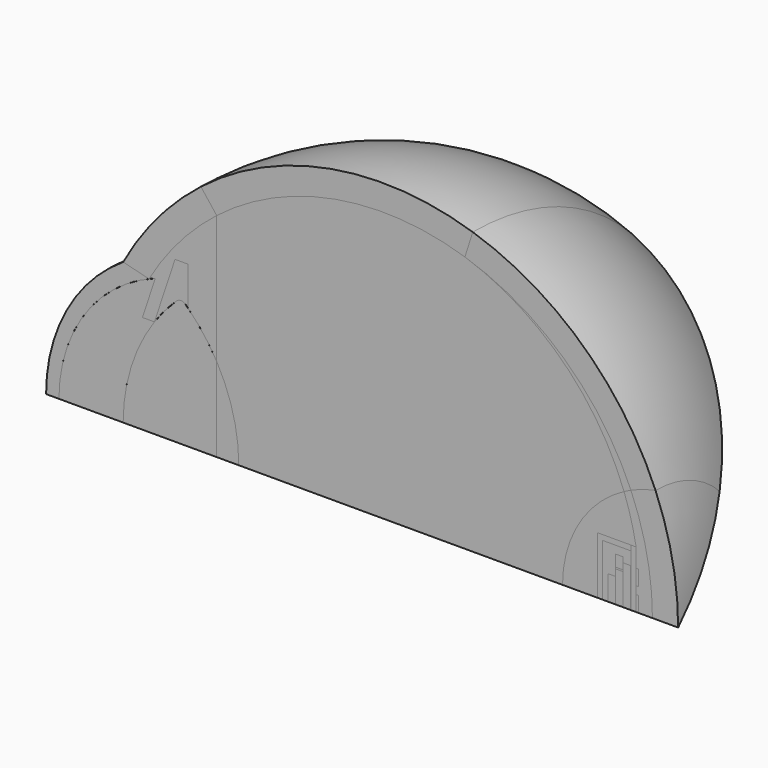
from build123d import *

# Parameters (mm, degrees)
F1_ANGLE  = 45
F3_ANGLE  = 45
F4_ANGLE  = 45
F6_ANGLE  = 45
F7_ANGLE  = 45
F9_ANGLE  = 45
F10_ANGLE = 45
F11_W     = 1.51221
F11_H     = 2.23
F12_ANGLE = 45
F13_ANGLE = 45
F15_ANGLE = 45
F16_ANGLE = 45
F19_ANGLE = 45
F22_ANGLE = 45
F25_ANGLE = 45
F28_ANGLE = 45
F31_ANGLE = 45
F34_ANGLE = 45
F35_W     = 0.19
F35_H     = 2.23
F36_ANGLE = 45
F37_W     = 0.19
F37_H     = 2.23
F38_ANGLE = 45
F40_ANGLE = 45
F41_ANGLE = 45
F42_W     = 0.3
F42_H     = 1.5222
F44_ANGLE = 45
F45_W     = 0.28
F45_H     = 1.2205
F47_ANGLE = 45
F48_W     = 0.301
F48_H     = 0.95912
F50_ANGLE = 45
F51_W     = 0.28
F51_H     = 0.447172
F53_ANGLE = 45
F54_W     = 0.025
F54_H     = 0.25075
F56_ANGLE = 45
F57_W     = 0.1
F57_H     = 0.6
F59_ANGLE = 45
F62_ANGLE = 45
F65_ANGLE = 45
F68_ANGLE = 45
F69_W     = 0.28
F69_H     = 0.06
F71_ANGLE = 45


with BuildPart() as f1:
    # F0 (on Front) → F1 (revolve)
    with BuildSketch(Plane.XZ):
        with BuildLine():
            Line((-11.5, 0), (11.5, 0))
            ThreePointArc((11.5, 0), (2.8377537956, 11.1443776585), (-10.0995049384, 5.5))
            ThreePointArc((-10.0995049384, 5.5), (-12.3007384778, 3.1324910215), (-13.0995049384, 0))
            Line((-13.0995049384, 0), (-11.5, 0))
        make_face()
    revolve(axis=Axis((0, 0, 0), (-1, 0, 0)), revolution_arc=F1_ANGLE)

    # F2 (on Front) → F3 (revolve, cut)
    with BuildSketch(Plane.XZ):
        with BuildLine():
            ThreePointArc((11.5, 0), (2.8377537956, 11.1443776585), (-10.0995049384, 5.5))
            Line((-10.0995049384, 5.5), (-9.0932667397, 5.25))
            ThreePointArc((-9.0932667397, 5.25), (2.7175999736, 10.142221176), (10.5, 0))
            Line((10.5, 0), (11.5, 0))
        make_face()
    revolve(axis=Axis((0, 0, 0), (-1, 0, 0)), revolution_arc=F3_ANGLE, mode=Mode.SUBTRACT)

    # F5 (on face) → F6 (revolve, cut)
    with BuildSketch(Plane.XZ):
        with BuildLine():
            ThreePointArc((-12.5995049384, 0), (-11.6423500551, 3.1565885979), (-9.0932667397, 5.25))
            Line((-9.0932667397, 5.25), (-10.0995049384, 5.5))
            ThreePointArc((-10.0995049384, 5.5), (-12.3007384778, 3.1324910215), (-13.0995049384, 0))
            Line((-13.0995049384, 0), (-12.5995049384, 0))
        make_face()
    revolve(axis=Axis((-12.2997524692, 0, 0), (-1, 0, 0)), revolution_arc=F6_ANGLE, mode=Mode.SUBTRACT)

    # F8 (on Front) → F9 (revolve, cut)
    with BuildSketch(Plane.XZ):
        with BuildLine():
            ThreePointArc((3.2015621187, 10), (8.2807192075, 6.1420955145), (10, 0))
            Line((10, 0), (10.5, 0))
            ThreePointArc((10.5, 0), (8.4813442993, 6.1900564518), (3.2015621187, 10))
        make_face()
    revolve(axis=Axis((0, 0, 0), (-1, 0, 0)), revolution_arc=F9_ANGLE, mode=Mode.SUBTRACT)

    # F11 (on face) → F12 (revolve, cut)
    with BuildSketch(Plane.XZ):
        with Locations((9.1086225685, 1.115)):
            Rectangle(F11_W, F11_H)
    revolve(axis=Axis((9.1086225685, 0, 0), (-1, 0, 0)), revolution_arc=F12_ANGLE, mode=Mode.SUBTRACT)

    # F14 (on Front) → F15 (revolve, cut)
    with BuildSketch(Plane.XZ):
        with BuildLine():
            ThreePointArc((10, 0), (9.9947523902, 1.1187845105), (9.8647275685, 2.23))
            Line((9.8647275685, 2.23), (9.8647275685, 0))
            Line((9.8647275685, 0), (10, 0))
        make_face()
    revolve(axis=Axis((9.9323637842, 0, 0), (-1, 0, 0)), revolution_arc=F15_ANGLE, mode=Mode.SUBTRACT)

    # F20 (on Front) → F21 (revolve, cut)
    with BuildSketch(Plane.XZ):
        with BuildLine():
            Line((-9.3495049384, 3.8445862413), (-8.8495049384, 5.3445862413))
            ThreePointArc((-8.8495049384, 5.3445862413), (-11.5684914777, 3.2644717065), (-12.5995049384, 0))
            Line((-12.5995049384, 0), (-8.8495049384, 0))
            Line((-8.8495049384, 0), (-8.8495049384, 3.8445862413))
            Line((-8.8495049384, 3.8445862413), (-9.3495049384, 3.8445862413))
        make_face()
    revolve(axis=Axis((-10.7245049384, 0, 0), (1, 0, 0)), mode=Mode.SUBTRACT)


with BuildPart() as f4:
    # F2 (on Front) → F4 (revolve)
    with BuildSketch(Plane.XZ):
        with BuildLine():
            ThreePointArc((11.5, 0), (2.8377537956, 11.1443776585), (-10.0995049384, 5.5))
            Line((-10.0995049384, 5.5), (-9.0932667397, 5.25))
            ThreePointArc((-9.0932667397, 5.25), (2.7175999736, 10.142221176), (10.5, 0))
            Line((10.5, 0), (11.5, 0))
        make_face()
    revolve(axis=Axis((0, 0, 0), (-1, 0, 0)), revolution_arc=F4_ANGLE)

    # F17 (on Front) → F18 (revolve, cut)
    with BuildSketch(Plane.XZ):
        with BuildLine():
            ThreePointArc((11.5, 0), (9.2890913754, 6.7795856377), (3.5064727967, 10.9523809524))
            Line((3.5064727967, 10.9523809524), (3.2015621187, 10))
            ThreePointArc((3.2015621187, 10), (8.4813442993, 6.1900564518), (10.5, 0))
            Line((10.5, 0), (11.5, 0))
        make_face()
    revolve(axis=Axis((11, 0, 0), (1, 0, 0)), mode=Mode.SUBTRACT)

    # F29 (on Front) → F30 (revolve, cut)
    with BuildSketch(Plane.XZ):
        with BuildLine():
            ThreePointArc((-9.0932667397, 5.25), (-7.9222484154, 6.8911523017), (-6.4591549508, 8.2782436134))
            Line((-6.4591549508, 8.2782436134), (-7.0743125651, 9.066647767))
            ThreePointArc((-7.0743125651, 9.066647767), (-8.7701337495, 7.438733361), (-10.0995049384, 5.5))
            Line((-10.0995049384, 5.5), (-9.0932667397, 5.25))
        make_face()
    revolve(axis=Axis((-7.8495049384, 0, 0), (-1, 0, 0)), mode=Mode.SUBTRACT)


with BuildPart() as f7:
    # F5 (on face) → F7 (revolve)
    with BuildSketch(Plane.XZ):
        with BuildLine():
            ThreePointArc((-12.5995049384, 0), (-11.6423500551, 3.1565885979), (-9.0932667397, 5.25))
            Line((-9.0932667397, 5.25), (-10.0995049384, 5.5))
            ThreePointArc((-10.0995049384, 5.5), (-12.3007384778, 3.1324910215), (-13.0995049384, 0))
            Line((-13.0995049384, 0), (-12.5995049384, 0))
        make_face()
    revolve(axis=Axis((0, 0, 0), (-1, 0, 0)), revolution_arc=F7_ANGLE)


with BuildPart() as f10:
    # F8 (on Front) → F10 (revolve)
    with BuildSketch(Plane.XZ):
        with BuildLine():
            ThreePointArc((3.2015621187, 10), (8.2807192075, 6.1420955145), (10, 0))
            Line((10, 0), (10.5, 0))
            ThreePointArc((10.5, 0), (8.4813442993, 6.1900564518), (3.2015621187, 10))
        make_face()
    revolve(axis=Axis((10.25, 0, 0), (-1, 0, 0)), revolution_arc=F10_ANGLE)


with BuildPart() as f13:
    # F11 (on face) → F13 (revolve)
    with BuildSketch(Plane.XZ):
        with Locations((9.1086225685, 1.115)):
            Rectangle(F11_W, F11_H)
    revolve(axis=Axis((0, 0, 0), (-1, 0, 0)), revolution_arc=F13_ANGLE)

    # F35 (on face) → F36 (revolve, cut)
    with BuildSketch(Plane.XZ):
        with Locations((9.7697275685, 1.115)):
            Rectangle(F35_W, F35_H)
    revolve(axis=Axis((0, 0, 0), (-1, 0, 0)), revolution_arc=F36_ANGLE, mode=Mode.SUBTRACT)

    # F39 (on face) → F40 (revolve, cut)
    with BuildSketch(Plane.XZ):
        Polygon((8.3525175685, 0), (8.5525175685, 0), (8.5525175685, 2.03), (9.6747275685, 2.03), (9.6747275685, 2.23), (8.3525175685, 2.23), align=None)
    revolve(axis=Axis((0, 0, 0), (-1, 0, 0)), revolution_arc=F40_ANGLE, mode=Mode.SUBTRACT)

    # F42 (on face) → F43 (revolve, cut)
    with BuildSketch(Plane.XZ):
        with Locations((9.4997275685, 0.7611)):
            Rectangle(F42_W, F42_H)
    revolve(axis=Axis((9.4997275685, 0, 0), (-1, 0, 0)), mode=Mode.SUBTRACT)

    # F45 (on face) → F46 (revolve, cut)
    with BuildSketch(Plane.XZ):
        with Locations((9.2097275685, 0.61025)):
            Rectangle(F45_W, F45_H)
    revolve(axis=Axis((9.2097275685, 0, 0), (-1, 0, 0)), mode=Mode.SUBTRACT)

    # F48 (on face) → F49 (revolve, cut)
    with BuildSketch(Plane.XZ):
        with Locations((8.9192275685, 0.47956)):
            Rectangle(F48_W, F48_H)
    revolve(axis=Axis((8.9192275685, 0, 0), (-1, 0, 0)), mode=Mode.SUBTRACT)

    # F51 (on face) → F52 (revolve, cut)
    with BuildSketch(Plane.XZ):
        with Locations((9.2097275685, 1.504086)):
            Rectangle(F51_W, F51_H)
    revolve(axis=Axis((0, 0, 0), (-1, 0, 0)), mode=Mode.SUBTRACT)

    # F54 (on face) → F55 (revolve, cut)
    with BuildSketch(Plane.XZ):
        with Locations((9.6622275685, 0.125375)):
            Rectangle(F54_W, F54_H)
        with Locations((9.6622275685, 1.125375)):
            Rectangle(F54_W, F54_H)
    revolve(axis=Axis((9.6622275685, 0, 0), (-1, 0, 0)), mode=Mode.SUBTRACT)

    # F69 (on face) → F70 (revolve, cut)
    with BuildSketch(Plane.XZ):
        with Locations((9.2097275685, 1.2505)):
            Rectangle(F69_W, F69_H)
    revolve(axis=Axis((0, 0, 0), (-1, 0, 0)), mode=Mode.SUBTRACT)


with BuildPart() as f16:
    # F14 (on Front) → F16 (revolve)
    with BuildSketch(Plane.XZ):
        with BuildLine():
            ThreePointArc((10, 0), (9.9947523902, 1.1187845105), (9.8647275685, 2.23))
            Line((9.8647275685, 2.23), (9.8647275685, 0))
            Line((9.8647275685, 0), (10, 0))
        make_face()
    revolve(axis=Axis((0, 0, 0), (-1, 0, 0)), revolution_arc=F16_ANGLE)


with BuildPart() as f19:
    # F17 (on Front) → F19 (revolve)
    with BuildSketch(Plane.XZ):
        with BuildLine():
            ThreePointArc((11.5, 0), (9.2890913754, 6.7795856377), (3.5064727967, 10.9523809524))
            Line((3.5064727967, 10.9523809524), (3.2015621187, 10))
            ThreePointArc((3.2015621187, 10), (8.4813442993, 6.1900564518), (10.5, 0))
            Line((10.5, 0), (11.5, 0))
        make_face()
    revolve(axis=Axis((0, 0, 0), (-1, 0, 0)), revolution_arc=F19_ANGLE)

    # F63 (on face) → F64 (revolve, cut)
    with BuildSketch(Plane.XZ):
        with BuildLine():
            ThreePointArc((11.5, 0), (11.2777435686, 2.25), (10.6195652174, 4.4130300921))
            ThreePointArc((10.6195652174, 4.4130300921), (10.1327706577, 4.2872699851), (9.6630434783, 4.1079910829))
            ThreePointArc((9.6630434783, 4.1079910829), (10.2886334496, 2.0961921999), (10.5, 0))
            Line((10.5, 0), (11.5, 0))
        make_face()
    revolve(axis=Axis((11, 0, 0), (-1, 0, 0)), mode=Mode.SUBTRACT)


with BuildPart() as f22:
    # F20 (on Front) → F22 (revolve)
    with BuildSketch(Plane.XZ):
        with BuildLine():
            Line((-9.3495049384, 3.8445862413), (-8.8495049384, 5.3445862413))
            ThreePointArc((-8.8495049384, 5.3445862413), (-11.5684914777, 3.2644717065), (-12.5995049384, 0))
            Line((-12.5995049384, 0), (-8.8495049384, 0))
            Line((-8.8495049384, 0), (-8.8495049384, 3.8445862413))
            Line((-8.8495049384, 3.8445862413), (-9.3495049384, 3.8445862413))
        make_face()
    revolve(axis=Axis((0, 0, 0), (-1, 0, 0)), revolution_arc=F22_ANGLE)


with BuildPart() as f24_tool:
    # F23 (on Front) → F24 (revolve)
    with BuildSketch(Plane.XZ):
        with BuildLine():
            Line((-10.0995049384, 0), (-5.5995049384, 0))
            ThreePointArc((-5.5995049384, 0), (-6.1408791354, 2.6344401261), (-7.6772587181, 4.8419044128))
            ThreePointArc((-7.6772587181, 4.8419044128), (-7.8495049384, 4.9107104847), (-8.0217511587, 4.8419044128))
            ThreePointArc((-8.0217511587, 4.8419044128), (-9.5581307413, 2.6344401261), (-10.0995049384, 0))
        make_face()
    revolve(axis=Axis((0, 0, 0), (-1, 0, 0)))


with BuildPart() as f1_1:
    add(f1.part)

    # F24: cut by f24_tool
    add(f24_tool.part, mode=Mode.SUBTRACT)

    # F26 (on Front) → F27 (revolve, cut)
    with BuildSketch(Plane.XZ):
        with BuildLine():
            Line((-8.8495049384, 5.3445862413), (-9.3495049384, 3.8445862413))
            Line((-9.3495049384, 3.8445862413), (-8.8823713109, 3.8445862413))
            Line((-8.8823713109, 3.8445862413), (-8.0810395972, 6.2485813822))
            Line((-8.0810395972, 6.2485813822), (-7.5810395972, 6.2485813822))
            Line((-7.5810395972, 6.2485813822), (-7.5810395972, 4.7485813822))
            ThreePointArc((-7.5810395972, 4.7485813822), (-6.9689696113, 4.0524234931), (-6.4591549508, 3.2782436134))
            Line((-6.4591549508, 3.2782436134), (-6.4591549508, 8.2782436134))
            ThreePointArc((-6.4591549508, 8.2782436134), (-7.9222484154, 6.8911523017), (-9.0932667397, 5.25))
            ThreePointArc((-9.0932667397, 5.25), (-8.9719298306, 5.298695062), (-8.8495049384, 5.3445862413))
        make_face()
    revolve(axis=Axis((-7.8495049384, 0, 0), (-1, 0, 0)), mode=Mode.SUBTRACT)

    # F60 (on face) → F61 (revolve, cut)
    with BuildSketch(Plane.XZ):
        with BuildLine():
            ThreePointArc((9.8647275685, 2.23), (9.6692210389, 3.1141957451), (9.3946322021, 3.9771128266))
            ThreePointArc((9.3946322021, 3.9771128266), (7.6448634855, 2.3211898791), (7, 0))
            Line((7, 0), (8.3525175685, 0))
            Line((8.3525175685, 0), (8.3525175685, 2.23))
            Line((8.3525175685, 2.23), (9.8647275685, 2.23))
        make_face()
    revolve(axis=Axis((7.6762587842, 0, 0), (1, 0, 0)), mode=Mode.SUBTRACT)


with BuildPart() as f22_1:
    add(f22.part)

    # F24: cut by f24_tool
    add(f24_tool.part, mode=Mode.SUBTRACT)


with BuildPart() as f25:
    # F23 (on Front) → F25 (revolve)
    with BuildSketch(Plane.XZ):
        with BuildLine():
            Line((-10.0995049384, 0), (-5.5995049384, 0))
            ThreePointArc((-5.5995049384, 0), (-6.1408791354, 2.6344401261), (-7.6772587181, 4.8419044128))
            ThreePointArc((-7.6772587181, 4.8419044128), (-7.8495049384, 4.9107104847), (-8.0217511587, 4.8419044128))
            ThreePointArc((-8.0217511587, 4.8419044128), (-9.5581307413, 2.6344401261), (-10.0995049384, 0))
        make_face()
    revolve(axis=Axis((0, 0, 0), (-1, 0, 0)), revolution_arc=F25_ANGLE)

    # F32 (on Front) → F33 (revolve, cut)
    with BuildSketch(Plane.XZ):
        with BuildLine():
            Line((-6.4591549508, 3.2782436134), (-6.4591549508, 0))
            Line((-6.4591549508, 0), (-5.5995049384, 0))
            ThreePointArc((-5.5995049384, 0), (-5.8179901834, 1.6945411866), (-6.4591549508, 3.2782436134))
        make_face()
    revolve(axis=Axis((-6.0293299446, 0, 0), (1, 0, 0)), mode=Mode.SUBTRACT)


with BuildPart() as f28:
    # F26 (on Front) → F28 (revolve)
    with BuildSketch(Plane.XZ):
        with BuildLine():
            Line((-8.8495049384, 5.3445862413), (-9.3495049384, 3.8445862413))
            Line((-9.3495049384, 3.8445862413), (-8.8823713109, 3.8445862413))
            Line((-8.8823713109, 3.8445862413), (-8.0810395972, 6.2485813822))
            Line((-8.0810395972, 6.2485813822), (-7.5810395972, 6.2485813822))
            Line((-7.5810395972, 6.2485813822), (-7.5810395972, 4.7485813822))
            ThreePointArc((-7.5810395972, 4.7485813822), (-6.9689696113, 4.0524234931), (-6.4591549508, 3.2782436134))
            Line((-6.4591549508, 3.2782436134), (-6.4591549508, 8.2782436134))
            ThreePointArc((-6.4591549508, 8.2782436134), (-7.9222484154, 6.8911523017), (-9.0932667397, 5.25))
            ThreePointArc((-9.0932667397, 5.25), (-8.9719298306, 5.298695062), (-8.8495049384, 5.3445862413))
        make_face()
    revolve(axis=Axis((-7.8495049384, 0, 0), (-1, 0, 0)), revolution_arc=F28_ANGLE)


with BuildPart() as f31:
    # F29 (on Front) → F31 (revolve)
    with BuildSketch(Plane.XZ):
        with BuildLine():
            ThreePointArc((-9.0932667397, 5.25), (-7.9222484154, 6.8911523017), (-6.4591549508, 8.2782436134))
            Line((-6.4591549508, 8.2782436134), (-7.0743125651, 9.066647767))
            ThreePointArc((-7.0743125651, 9.066647767), (-8.7701337495, 7.438733361), (-10.0995049384, 5.5))
            Line((-10.0995049384, 5.5), (-9.0932667397, 5.25))
        make_face()
    revolve(axis=Axis((-7.8495049384, 0, 0), (-1, 0, 0)), revolution_arc=F31_ANGLE)


with BuildPart() as f34:
    # F32 (on Front) → F34 (revolve)
    with BuildSketch(Plane.XZ):
        with BuildLine():
            Line((-6.4591549508, 3.2782436134), (-6.4591549508, 0))
            Line((-6.4591549508, 0), (-5.5995049384, 0))
            ThreePointArc((-5.5995049384, 0), (-5.8179901834, 1.6945411866), (-6.4591549508, 3.2782436134))
        make_face()
    revolve(axis=Axis((-7.8495049384, 0, 0), (-1, 0, 0)), revolution_arc=F34_ANGLE)


with BuildPart() as f38:
    # F37 (on face) → F38 (revolve)
    with BuildSketch(Plane.XZ):
        with Locations((9.7697275685, 1.115)):
            Rectangle(F37_W, F37_H)
    revolve(axis=Axis((0, 0, 0), (-1, 0, 0)), revolution_arc=F38_ANGLE)


with BuildPart() as f41:
    # F39 (on face) → F41 (revolve)
    with BuildSketch(Plane.XZ):
        Polygon((8.3525175685, 0), (8.5525175685, 0), (8.5525175685, 2.03), (9.6747275685, 2.03), (9.6747275685, 2.23), (8.3525175685, 2.23), align=None)
    revolve(axis=Axis((0, 0, 0), (-1, 0, 0)), revolution_arc=F41_ANGLE)


with BuildPart() as f44:
    # F42 (on face) → F44 (revolve)
    with BuildSketch(Plane.XZ):
        with Locations((9.4997275685, 0.7611)):
            Rectangle(F42_W, F42_H)
    revolve(axis=Axis((0, 0, 0), (-1, 0, 0)), revolution_arc=F44_ANGLE)


with BuildPart() as f47:
    # F45 (on face) → F47 (revolve)
    with BuildSketch(Plane.XZ):
        with Locations((9.2097275685, 0.61025)):
            Rectangle(F45_W, F45_H)
    revolve(axis=Axis((0, 0, 0), (-1, 0, 0)), revolution_arc=F47_ANGLE)


with BuildPart() as f50:
    # F48 (on face) → F50 (revolve)
    with BuildSketch(Plane.XZ):
        with Locations((8.9192275685, 0.47956)):
            Rectangle(F48_W, F48_H)
    revolve(axis=Axis((0, 0, 0), (-1, 0, 0)), revolution_arc=F50_ANGLE)


with BuildPart() as f53:
    # F51 (on face) → F53 (revolve)
    with BuildSketch(Plane.XZ):
        with Locations((9.2097275685, 1.504086)):
            Rectangle(F51_W, F51_H)
    revolve(axis=Axis((0, 0, 0), (-1, 0, 0)), revolution_arc=F53_ANGLE)


with BuildPart() as f56:
    # F54 (on face) → F56 (revolve)
    with BuildSketch(Plane.XZ):
        with Locations((9.6622275685, 0.125375)):
            Rectangle(F54_W, F54_H)
    revolve(axis=Axis((0, 0, 0), (-1, 0, 0)), revolution_arc=F56_ANGLE)


with BuildPart() as f56b:
    # F54 (on face) → F56, piece 2 (revolve)
    with BuildSketch(Plane.XZ):
        with Locations((9.6622275685, 1.125375)):
            Rectangle(F54_W, F54_H)
    revolve(axis=Axis((0, 0, 0), (-1, 0, 0)), revolution_arc=F56_ANGLE)


with BuildPart() as f58_tool:
    # F57 (on face) → F58 (revolve)
    with BuildSketch(Plane.XZ):
        with Locations((9.9147275685, 0.3)):
            Rectangle(F57_W, F57_H)
        with Locations((9.9147275685, 1.2)):
            Rectangle(F57_W, F57_H)
    revolve(axis=Axis((9.9147275685, 0, 0), (1, 0, 0)))


with BuildPart() as f10_1:
    add(f10.part)

    # F58: cut by f58_tool
    add(f58_tool.part, mode=Mode.SUBTRACT)


with BuildPart() as f16_1:
    add(f16.part)

    # F58: cut by f58_tool
    add(f58_tool.part, mode=Mode.SUBTRACT)


with BuildPart() as f59:
    # F57 (on face) → F59 (revolve)
    with BuildSketch(Plane.XZ):
        with Locations((9.9147275685, 0.3)):
            Rectangle(F57_W, F57_H)
    revolve(axis=Axis((0, 0, 0), (-1, 0, 0)), revolution_arc=F59_ANGLE)


with BuildPart() as f59b:
    # F57 (on face) → F59, piece 2 (revolve)
    with BuildSketch(Plane.XZ):
        with Locations((9.9147275685, 1.2)):
            Rectangle(F57_W, F57_H)
    revolve(axis=Axis((0, 0, 0), (-1, 0, 0)), revolution_arc=F59_ANGLE)


with BuildPart() as f62:
    # F60 (on face) → F62 (revolve)
    with BuildSketch(Plane.XZ):
        with BuildLine():
            ThreePointArc((9.8647275685, 2.23), (9.6692210389, 3.1141957451), (9.3946322021, 3.9771128266))
            ThreePointArc((9.3946322021, 3.9771128266), (7.6448634855, 2.3211898791), (7, 0))
            Line((7, 0), (8.3525175685, 0))
            Line((8.3525175685, 0), (8.3525175685, 2.23))
            Line((8.3525175685, 2.23), (9.8647275685, 2.23))
        make_face()
    revolve(axis=Axis((0, 0, 0), (-1, 0, 0)), revolution_arc=F62_ANGLE)


with BuildPart() as f65:
    # F63 (on face) → F65 (revolve)
    with BuildSketch(Plane.XZ):
        with BuildLine():
            ThreePointArc((11.5, 0), (11.2777435686, 2.25), (10.6195652174, 4.4130300921))
            ThreePointArc((10.6195652174, 4.4130300921), (10.1327706577, 4.2872699851), (9.6630434783, 4.1079910829))
            ThreePointArc((9.6630434783, 4.1079910829), (10.2886334496, 2.0961921999), (10.5, 0))
            Line((10.5, 0), (11.5, 0))
        make_face()
    revolve(axis=Axis((0, 0, 0), (-1, 0, 0)), revolution_arc=F65_ANGLE)


with BuildPart() as f67_tool:
    # F66 (on face) → F67 (revolve)
    with BuildSketch(Plane.XZ):
        with BuildLine():
            ThreePointArc((10.5, 0), (10.2886334496, 2.0961921999), (9.6630434783, 4.1079910829))
            ThreePointArc((9.6630434783, 4.1079910829), (9.5277519071, 4.0447790372), (9.3946322021, 3.9771128266))
            ThreePointArc((9.3946322021, 3.9771128266), (9.6692210389, 3.1141957451), (9.8647275685, 2.23))
            Line((9.8647275685, 2.23), (9.8647275685, 1.5))
            Line((9.8647275685, 1.5), (9.9647275685, 1.5))
            Line((9.9647275685, 1.5), (9.9647275685, 0.9))
            Line((9.9647275685, 0.9), (9.8647275685, 0.9))
            Line((9.8647275685, 0.9), (9.8647275685, 0.6))
            Line((9.8647275685, 0.6), (9.9647275685, 0.6))
            Line((9.9647275685, 0.6), (9.9647275685, 0))
            Line((9.9647275685, 0), (10.5, 0))
        make_face()
    revolve(axis=Axis((10.2323637842, 0, 0), (-1, 0, 0)))


with BuildPart() as f10_2:
    add(f10_1.part)

    # F67: cut by f67_tool
    add(f67_tool.part, mode=Mode.SUBTRACT)


with BuildPart() as f16_2:
    add(f16_1.part)

    # F67: cut by f67_tool
    add(f67_tool.part, mode=Mode.SUBTRACT)


with BuildPart() as f68:
    # F66 (on face) → F68 (revolve)
    with BuildSketch(Plane.XZ):
        with BuildLine():
            ThreePointArc((10.5, 0), (10.2886334496, 2.0961921999), (9.6630434783, 4.1079910829))
            ThreePointArc((9.6630434783, 4.1079910829), (9.5277519071, 4.0447790372), (9.3946322021, 3.9771128266))
            ThreePointArc((9.3946322021, 3.9771128266), (9.6692210389, 3.1141957451), (9.8647275685, 2.23))
            Line((9.8647275685, 2.23), (9.8647275685, 1.5))
            Line((9.8647275685, 1.5), (9.9647275685, 1.5))
            Line((9.9647275685, 1.5), (9.9647275685, 0.9))
            Line((9.9647275685, 0.9), (9.8647275685, 0.9))
            Line((9.8647275685, 0.9), (9.8647275685, 0.6))
            Line((9.8647275685, 0.6), (9.9647275685, 0.6))
            Line((9.9647275685, 0.6), (9.9647275685, 0))
            Line((9.9647275685, 0), (10.5, 0))
        make_face()
    revolve(axis=Axis((0, 0, 0), (-1, 0, 0)), revolution_arc=F68_ANGLE)


with BuildPart() as f71:
    # F69 (on face) → F71 (revolve)
    with BuildSketch(Plane.XZ):
        with Locations((9.2097275685, 1.2505)):
            Rectangle(F69_W, F69_H)
    revolve(axis=Axis((0, 0, 0), (-1, 0, 0)), revolution_arc=F71_ANGLE)


solid = Compound([f4.part, f7.part, f13.part, f19.part, f1_1.part, f22_1.part, f25.part, f28.part, f31.part, f34.part, f38.part, f41.part, f44.part, f47.part, f50.part, f53.part, f56.part, f56b.part, f59.part, f59b.part, f62.part, f65.part, f10_2.part, f68.part, f71.part])
